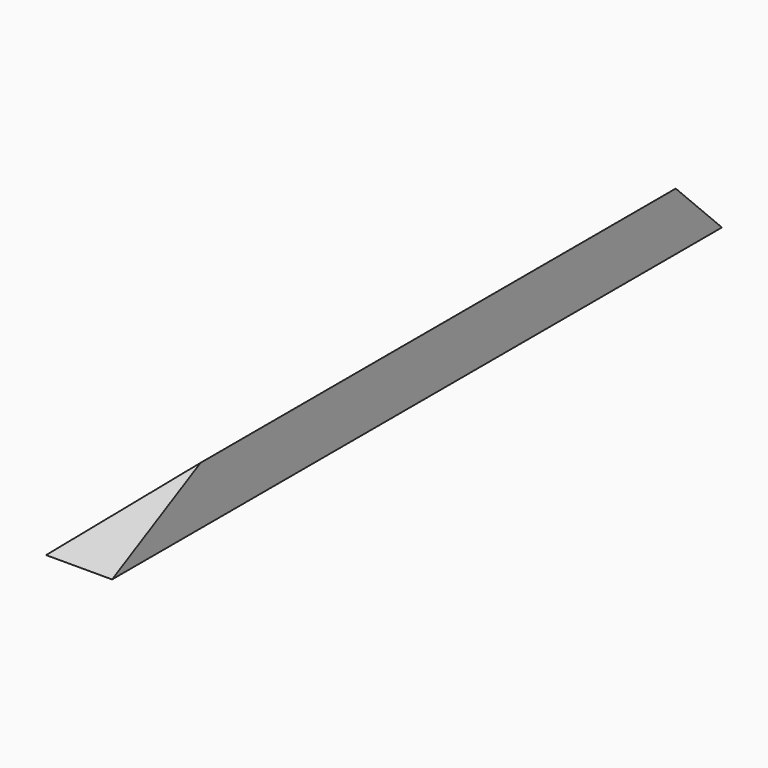
from build123d import *

# Parameters (mm, degrees)
F0_W     = 20
F0_H     = 231
F1_DEPTH = 8.75
F2_SIZE2 = 17.49999
F2_SIZE  = 33.49999
F3_SIZE2 = 17.49999
F3_SIZE  = 17.49999
F4_SIZE2 = 17.49999
F4_SIZE  = 19.99999


# Not quite as in the source:
# - a fillet or chamfer is up to 0.001 mm smaller than in the source, because OpenCascade refuses the exact size


with BuildPart() as f1:
    # F0 (on Top) → F1 (new body, symmetric)
    with BuildSketch(Plane.XY):
        Rectangle(F0_W, F0_H)
    extrude(amount=F1_DEPTH, both=True)

    # F2 (size 33.5 and 17.5 in the source; OpenCascade refuses exactly that, so slightly less here)
    f2_edges = [f1.edges().sort_by_distance(p)[0] for p in [
        (0, -115.5, 8.75),
    ]]
    f2_side = f1.faces().sort_by_distance((0, 0, 8.75))[0]
    chamfer(f2_edges, length=F2_SIZE, length2=F2_SIZE2, reference=f2_side)

    # F3 (size 17.5 and 17.5 in the source; OpenCascade refuses exactly that, so slightly less here)
    f3_edges = [f1.edges().sort_by_distance(p)[0] for p in [
        (0, 115.5, 8.75),
    ]]
    chamfer(f3_edges, length=F3_SIZE, length2=F3_SIZE2)

    # F4 (size 20 and 17.5 in the source; OpenCascade refuses exactly that, so slightly less here)
    f4_edges = [f1.edges().sort_by_distance(p)[0] for p in [
        (-10, 8, 8.75),
    ]]
    f4_side = f1.faces().sort_by_distance((0, 8, 8.75))[0]
    chamfer(f4_edges, length=F4_SIZE, length2=F4_SIZE2, reference=f4_side)


solid = f1.part
